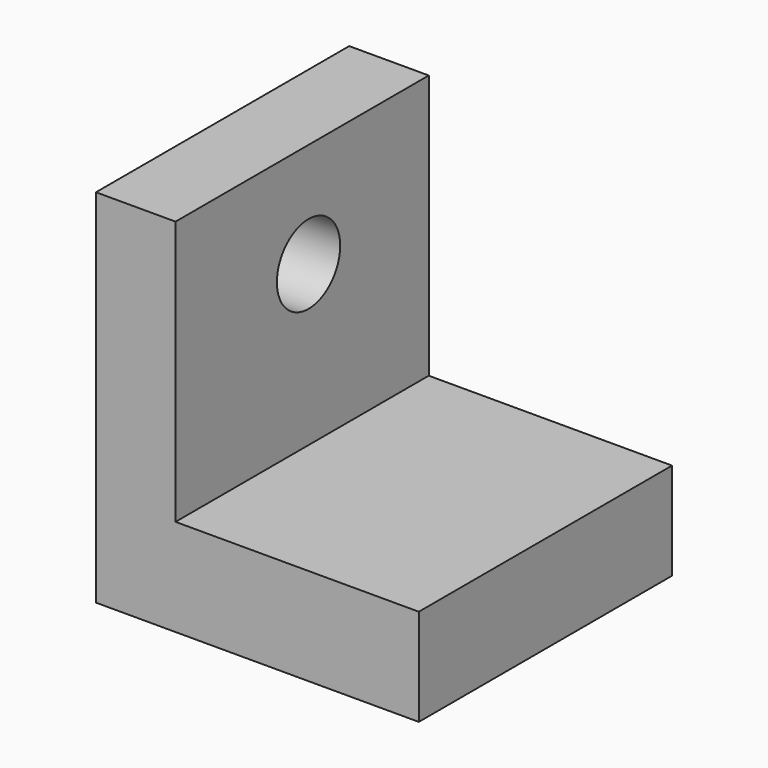
from build123d import *

# Parameters (mm, degrees)
F0_W     = 51.813559141
F0_H     = 32.5880763121
F1_DEPTH = 25.4
F2_DEPTH = 25.4
F3_DEPTH = 25.4
F4_DEPTH = 7.1882
F6_DEPTH = 37.846
F7_R     = 6.35
F8_DEPTH = 50.8
F9_DEPTH = 4.572


# Not quite as in the source:
# - a feature of the source that left no trace in its solid (it failed there, or was rolled back) is left out


with BuildPart() as f1:
    # F0 (on Front) → F1 (new body)
    with BuildSketch(Plane.XZ):
        with Locations((-23.6830220092, 10.7818876859)):
            Rectangle(F0_W, F0_H)
    extrude(amount=F1_DEPTH)

    # F2 (add): a face of the model
    f2_faces = [f1.faces().sort_by_distance(p)[0] for p in [
        (-23.6830220092, -25.4, 10.7818876859),
    ]]
    extrude(f2_faces, amount=F2_DEPTH)

    # F3 (add): a face of the model
    f3_faces = [f1.faces().sort_by_distance(p)[0] for p in [
        (-23.6830220092, -25.4, 27.0759258419),
    ]]
    extrude(f3_faces, amount=F3_DEPTH)

    # F4 (add): a face of the model
    f4_faces = [f1.faces().sort_by_distance(p)[0] for p in [
        (-23.6830220092, -25.4, 52.4759258419),
    ]]
    extrude(f4_faces, amount=-F4_DEPTH)

    # F5 (on face) → F6 (cut)
    with BuildSketch(Plane.XY.offset(52.4759258419)):
        Polygon((-36.8200466037, 0), (-36.8200466037, -25.4), (-36.8200466037, -50.8), (2.2237575613, -50.8), (2.2237575613, 0), align=None)
    extrude(amount=-F6_DEPTH, mode=Mode.SUBTRACT)

    # F7 (on face) → F8 (cut)
    with BuildSketch(Plane.YZ.offset(-36.8200466037)):
        with Locations((-24.1173226386, 35.6486514211)):
            Circle(F7_R)
    extrude(amount=-F8_DEPTH, mode=Mode.SUBTRACT)

    # F9 (cut): a face of the model
    f9_faces = [f1.faces().sort_by_distance(p)[0] for p in [
        (-17.2981445212, -25.4, 14.6299258419),
    ]]
    extrude(f9_faces, amount=-F9_DEPTH, mode=Mode.SUBTRACT)


solid = f1.part
